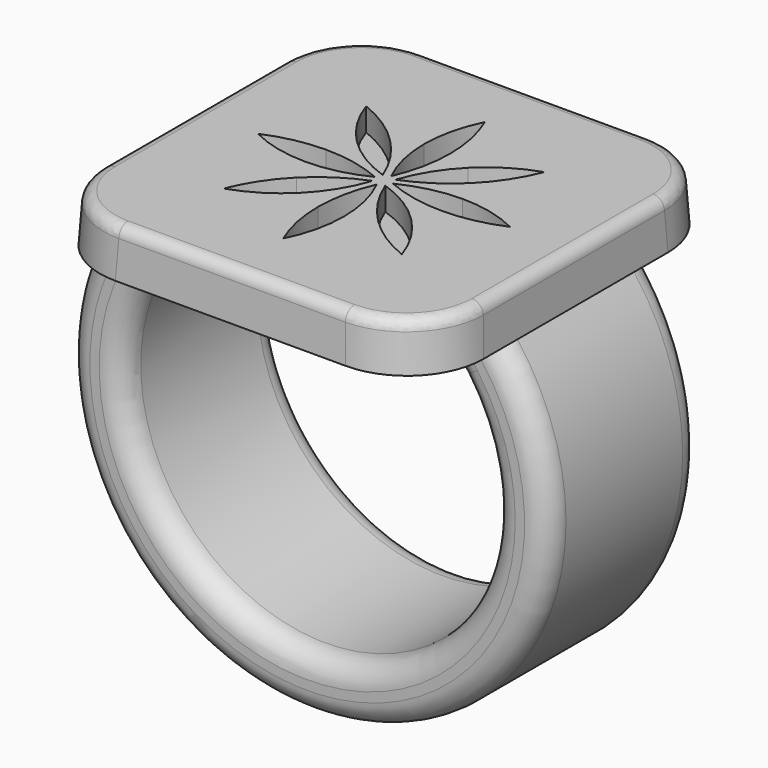
from build123d import *

# Parameters (mm, degrees)
F0_W          = 25.4
F0_H          = 25.4
F1_DEPTH      = 3.175
F1_TAPER      = 3
F3_W          = 5.08
F3_H          = 12.7
F6_DEPTH      = 6.35
F6_DEPTH_BACK = 6.35
F7_R          = 5.08
F8_R          = 1.524
F9_R          = 0.762
F11_DEPTH     = 1.524


# Not quite as in the source:
# - ends of sketch curves that miss each other by under 0.0002 mm in the source are joined


with BuildPart() as f1:
    # F0 (on Top) → F1 (new body)
    with BuildSketch(Plane.XY):
        Rectangle(F0_W, F0_H)
    extrude(amount=F1_DEPTH, taper=F1_TAPER)

    # F4: sweep along a path in F2
    with BuildLine(Plane.XZ) as f4_path:
        ThreePointArc((-10.16, 0), (0, -23.5582897328), (10.16, 0))
    # F3 (on face) → F4 (sweep)
    with BuildSketch(Plane(origin=(0, 0, 0), x_dir=(1, 0, 0), z_dir=(0, 0, -1))):
        with Locations((-10.16, 0)):
            Rectangle(F3_W, F3_H)
    sweep(path=f4_path.line)

    # F5 (on Front) → F6 (join, two sides)
    with BuildSketch(Plane.XZ) as f6_sk:
        with BuildLine():
            Line((10.0130578512, -2.535746045), (10.16, 0))
            Line((10.16, 0), (7.62, 0))
            ThreePointArc((7.62, 0), (8.9072265211, -1.1822790439), (10.0130578512, -2.535746045))
        make_face()
    extrude(amount=F6_DEPTH)
    extrude(f6_sk.sketch, amount=-F6_DEPTH_BACK)

    # F7
    f7_edges = [f1.edges().sort_by_distance(p)[0] for p in [
        (-12.616803, 12.616803, 1.5875),
        (12.616803, 12.616803, 1.5875),
        (12.616803, -12.616803, 1.5875),
        (-12.616803, -12.616803, 1.5875),
    ]]
    fillet(f7_edges, radius=F7_R)

    # F8
    f8_edges = [f1.edges().sort_by_distance(p)[0] for p in [
        (-1.743325, -6.35, -21.711017),
        (8.907227, -6.35, -1.182279),
        (-1.743325, 6.35, -21.711017),
        (0, -6.35, -25.501344),
        (0, 6.35, -25.501344),
        (8.907227, 6.35, -1.182279),
    ]]
    fillet(f8_edges, radius=F8_R)

    # F9
    f9_edges = [f1.edges().sort_by_distance(p)[0] for p in [
        (12.533605, 0, 3.175),
        (11.048589, -11.048589, 3.175),
        (11.048589, 11.048589, 3.175),
        (0, -12.533605, 3.175),
        (0, 12.533605, 3.175),
        (-11.048589, -11.048589, 3.175),
        (-11.048589, 11.048589, 3.175),
        (-12.533605, 0, 3.175),
    ]]
    fillet(f9_edges, radius=F9_R)

    # F10 (on face) → F11 (cut)
    with BuildSketch(Plane.XY.offset(3.175)):
        with BuildLine():
            ThreePointArc((-0.9155201148, 4.4694258476), (-0.6832986187, 2.4793758179), (3.5409e-06, 0.595941693))
            ThreePointArc((3.5409e-06, 0.595941693), (0.6027711391, 2.4909604976), (0.8062465423, 4.4690792099))
            ThreePointArc((0.8062465423, 4.4690792099), (0.6018941572, 6.4474337167), (-0.0016602711, 8.3425243592))
            ThreePointArc((-0.0016602711, 8.3425243592), (-0.6841903658, 6.4592148863), (-0.9155201148, 4.4694258476))
        make_face()
        with BuildLine():
            ThreePointArc((-3.8077546959, 2.5130013299), (-2.2363761453, 1.2700310995), (-0.42142512, 0.4214096769))
            ThreePointArc((-0.42142512, 0.4214096769), (-1.3351515877, 2.1875999181), (-2.5900116585, 3.730219495))
            ThreePointArc((-2.5900116585, 3.730219495), (-4.1334248315, 4.984630209), (-5.9002408115, 5.8978835339))
            ThreePointArc((-5.9002408115, 5.8978835339), (-5.0511485615, 4.0835502168), (-3.8077546959, 2.5130013299))
        make_face()
        with BuildLine():
            ThreePointArc((-4.4694348001, -0.9155173616), (-2.4793902981, -0.6832971735), (-0.5959608043, 1.2077e-06))
            ThreePointArc((-0.5959608043, 1.2077e-06), (-2.4909447448, 0.6027830722), (-4.4690604127, 0.8062578417))
            ThreePointArc((-4.4690604127, 0.8062578417), (-6.4474325455, 0.601904437), (-8.3425275239, -0.00165301))
            ThreePointArc((-8.3425275239, -0.00165301), (-6.4592135153, -0.6841876238), (-4.4694348001, -0.9155173616))
        make_face()
        with BuildLine():
            ThreePointArc((-2.5129958106, -3.8077433876), (-1.2700192482, -2.2363545852), (-0.4213965439, -0.4213909469))
            ThreePointArc((-0.4213965439, -0.4213909469), (-2.1876007302, -1.3351301119), (-3.7302203071, -2.5899901827))
            ThreePointArc((-3.7302203071, -2.5899901827), (-4.9846026422, -4.1333687575), (-5.8978587184, -5.9001801375))
            ThreePointArc((-5.8978587184, -5.9001801375), (-4.0835524313, -5.0511464123), (-2.5129958106, -3.8077433876))
        make_face()
        with BuildLine():
            ThreePointArc((0.9155173616, -4.4694348001), (0.6832945611, -2.4793792452), (-1.13725e-05, -0.5959404907))
            ThreePointArc((-1.13725e-05, -0.5959404907), (-0.6027958982, -2.4909317217), (-0.8062773019, -4.4690538311))
            ThreePointArc((-0.8062773019, -4.4690538311), (-0.6019215796, -6.4474219971), (0.0016427937, -8.3425269237))
            ThreePointArc((0.0016427937, -8.3425269237), (0.6841820315, -6.4592115317), (0.9155173616, -4.4694348001))
        make_face()
        with BuildLine():
            ThreePointArc((3.8077560876, -2.5129831047), (2.2363622238, -1.2699985662), (0.4213909469, -0.4213711439))
            ThreePointArc((0.4213909469, -0.4213711439), (1.3351322844, -2.1875874429), (2.5899988338, -3.7302169049))
            ThreePointArc((2.5899988338, -3.7302169049), (4.1334023383, -4.9846239173), (5.9002137183, -5.8978799935))
            ThreePointArc((5.9002137183, -5.8978799935), (5.0511591496, -4.083539721), (3.8077560876, -2.5129831047))
        make_face()
        with BuildLine():
            ThreePointArc((4.4694176698, 0.9155360845), (2.4793565872, 0.6833119761), (0.5959132016, 2.2641e-06))
            ThreePointArc((0.5959132016, 2.2641e-06), (2.4909366376, -0.6027661111), (4.4690537829, -0.8062464814))
            ThreePointArc((4.4690537829, -0.8062464814), (6.4474197136, -0.6018917801), (8.3425203043, 0.0016695744))
            ThreePointArc((8.3425203043, 0.0016695744), (6.4592208932, 0.6842008215), (4.4694176698, 0.9155360845))
        make_face()
        with BuildLine():
            ThreePointArc((2.5129838216, 3.8077483112), (1.2700056151, 2.2363646991), (0.4213794744, 0.4214060353))
            ThreePointArc((0.4213794744, 0.4214060353), (2.1875900431, 1.3351451192), (3.7302195051, 2.5900116686))
            ThreePointArc((3.7302195051, 2.5900116686), (4.984630209, 4.1334248315), (5.8978835339, 5.9002408115))
            ThreePointArc((5.8978835339, 5.9002408115), (4.0835473797, 5.0511570071), (2.5129838216, 3.8077483112))
        make_face()
    extrude(amount=-F11_DEPTH, mode=Mode.SUBTRACT)


solid = f1.part
